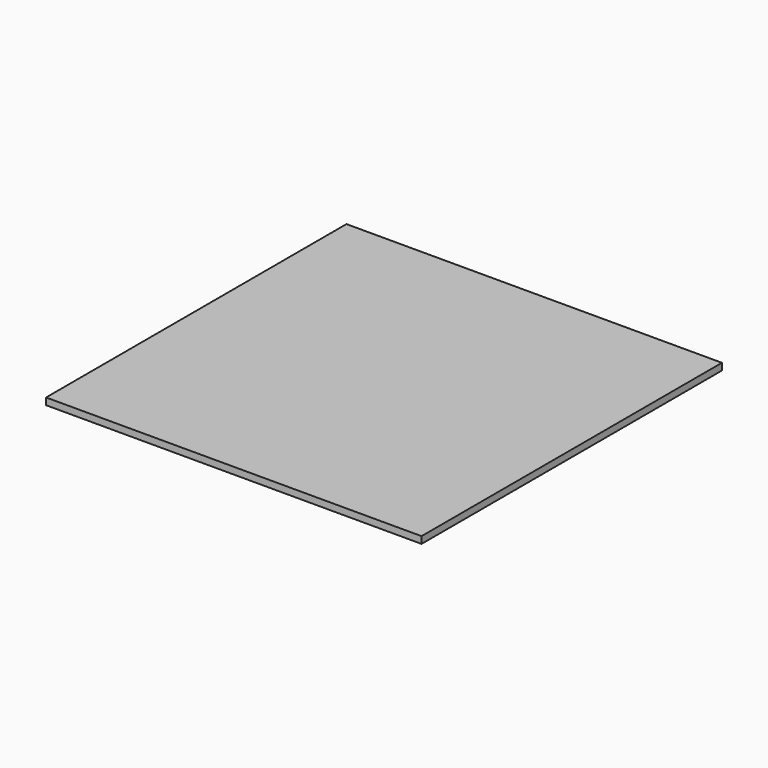
from build123d import *

# Parameters (mm, degrees)
F0_W     = 609.6
F0_H     = 609.6
F1_DEPTH = 11.1125


# Not quite as in the source:
# - a length typed as a fraction of an inch, garbled in the dataset ("3 / 203.2 mm" for 3/8 in), is restored


with BuildPart() as f1:
    # F0 (on Top) → F1 (new body)
    with BuildSketch(Plane.XY):
        Rectangle(F0_W, F0_H)
    extrude(amount=F1_DEPTH)


solid = f1.part
